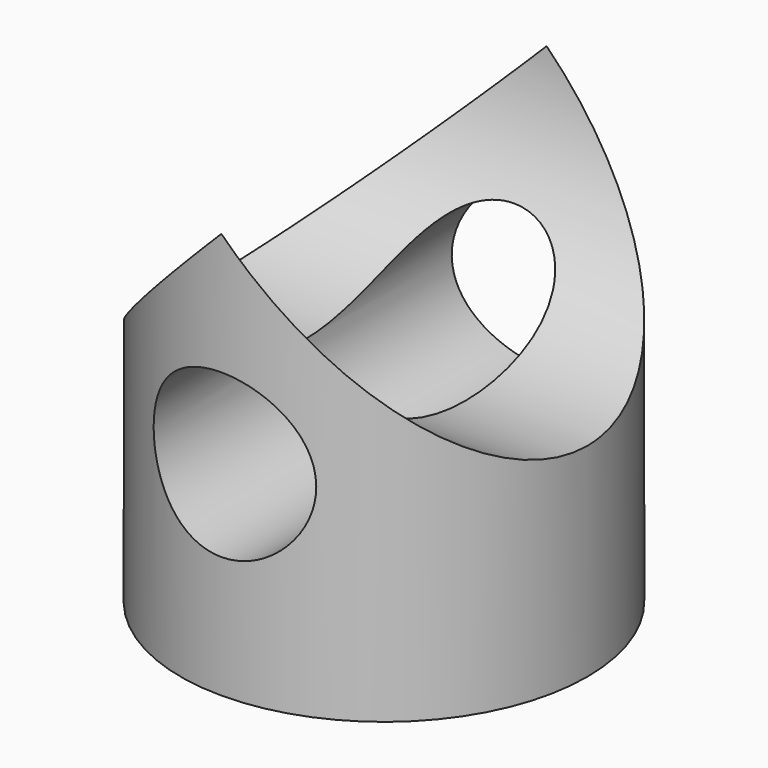
from build123d import *

# Parameters (mm, degrees)
F0_R          = 25
F1_DEPTH      = 50
F3_DEPTH      = 25.001
F3_DEPTH_BACK = 25.001
F4_R          = 10
F5_DEPTH      = 25.001
F5_DEPTH_BACK = 25.001


with BuildPart() as f1:
    # F0 (on Top) → F1 (new body)
    with BuildSketch(Plane.XY):
        Circle(F0_R)
    extrude(amount=F1_DEPTH)

    # F2 (on Right) → F3 (cut, two sides)
    with BuildSketch(Plane.YZ) as f3_sk:
        with BuildLine():
            ThreePointArc((-25, 50), (0, 25), (25, 50))
            ThreePointArc((25, 50), (0, 75), (-25, 50))
        make_face()
    extrude(amount=-F3_DEPTH, mode=Mode.SUBTRACT)
    extrude(f3_sk.sketch, amount=F3_DEPTH_BACK, mode=Mode.SUBTRACT)

    # F4 (on Front) → F5 (cut, two sides)
    with BuildSketch(Plane.XZ) as f5_sk:
        with Locations((0, 25)):
            Circle(F4_R)
    extrude(amount=F5_DEPTH, mode=Mode.SUBTRACT)
    extrude(f5_sk.sketch, amount=-F5_DEPTH_BACK, mode=Mode.SUBTRACT)


solid = f1.part
